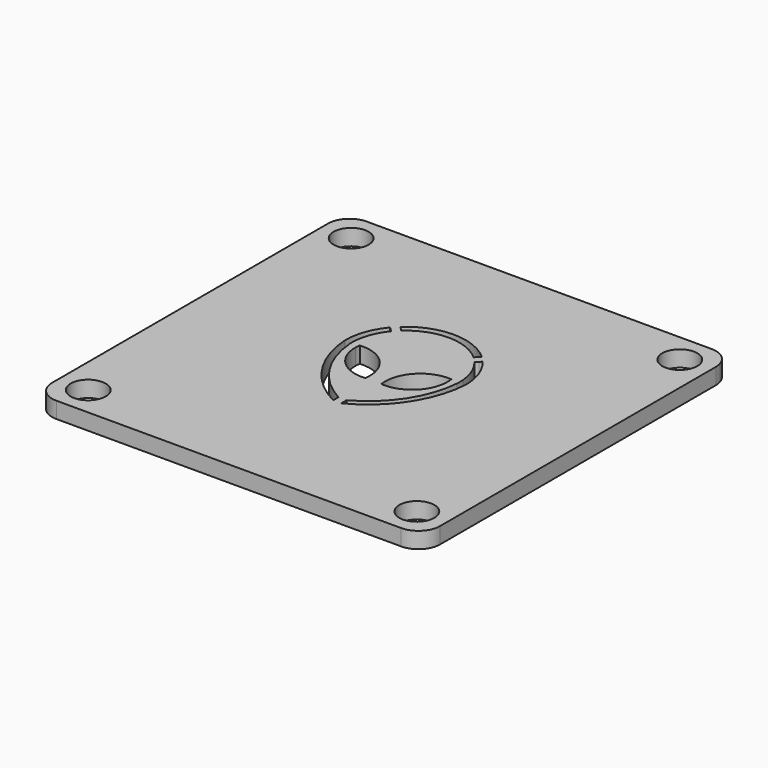
from build123d import *

# Parameters (mm, degrees)
F0_W        = 36
F0_H        = 36
F0_R        = 1.625
F1_DEPTH    = 1.5
F2_R        = 2
F3_T1_DEPTH = 3.5843159378
F3_T3_DEPTH = 3.5765382717


# Not quite as in the source:
# - a fillet or chamfer that OpenCascade refuses, or shapes differently, is made with other operations: its cross-section is extruded or revolved along the edge and cut away or added


with BuildPart() as f1:
    # F0 (on Top) → F1 (new body)
    with BuildSketch(Plane.XY):
        with Locations((18, -18)):
            Rectangle(F0_W, F0_H)
        with Locations((2.75, -33.25)):
            Circle(F0_R, mode=Mode.SUBTRACT)
        with Locations((33.25, -33.25)):
            Circle(F0_R, mode=Mode.SUBTRACT)
        with BuildLine():
            ThreePointArc((21.7779175478, -11.3763919814), (22.046238649, -11.6387988402), (22.2963811606, -11.918588577))
            ThreePointArc((22.2963811606, -11.918588577), (23.2607600241, -13.5926773143), (23.5988556823, -15.4948579101))
            ThreePointArc((23.5988556823, -15.4948579101), (22.0425607669, -20.1541714045), (18.3719356765, -23.4187950503))
            ThreePointArc((18.3719356765, -23.4187950503), (18.1854087753, -23.510113363), (17.9969356765, -23.5973441498))
            ThreePointArc((17.9969356765, -23.5973441498), (17.8078713111, -23.5092095417), (17.6207740645, -23.4169725439))
            ThreePointArc((17.6207740645, -23.4169725439), (13.9590716003, -20.150973111), (12.3987158352, -15.4990802577))
            ThreePointArc((12.3987158352, -15.4990802577), (12.7360960776, -13.5946679159), (13.7011902766, -11.9185996051))
            ThreePointArc((13.7011902766, -11.9185996051), (13.9513320879, -11.638809208), (14.2196525358, -11.3764016446))
            ThreePointArc((14.2196525358, -11.3764016446), (17.9987831657, -9.9089991809), (21.7779175478, -11.3763919814))
        make_face(mode=Mode.SUBTRACT)
        with Locations((2.75, -2.75)):
            Circle(F0_R, mode=Mode.SUBTRACT)
        with Locations((33.25, -2.75)):
            Circle(F0_R, mode=Mode.SUBTRACT)
        with BuildLine():
            ThreePointArc((18.3719356765, -22.8064015707), (21.6418869825, -19.7559203536), (22.9988556823, -15.4948579101))
            ThreePointArc((22.9988556823, -15.4948579101), (22.7058670076, -13.8225937813), (21.8702080342, -12.3447630196))
            ThreePointArc((21.8702080342, -12.3447630196), (21.6219028277, -12.0632376766), (21.3531767506, -11.8011340904))
            ThreePointArc((21.3531767506, -11.8011340904), (17.9987795183, -10.508999181), (14.644381672, -11.8011324963))
            ThreePointArc((14.644381672, -11.8011324963), (14.3756554704, -12.0632359548), (14.12735013, -12.3447611798))
            ThreePointArc((14.12735013, -12.3447611798), (13.2916900536, -13.8225926629), (12.9987009782, -15.4948579101))
            ThreePointArc((12.9987009782, -15.4948579101), (14.3541308063, -19.7551514484), (17.6219356765, -22.8061746181))
            ThreePointArc((17.6219356765, -22.8061746181), (17.8082968783, -22.9039932616), (17.9969356765, -22.9973441498))
            ThreePointArc((17.9969356765, -22.9973441498), (18.1855728443, -22.9041061909), (18.3719356765, -22.8064015707))
        make_face()
        with BuildLine():
            ThreePointArc((13.7508900496, -15.5000002377), (16.4147091349, -16.5221024247), (17.2508900496, -19.2500002377))
            ThreePointArc((17.2508900496, -19.2500002377), (14.7355024037, -18.3769724477), (13.7124911572, -15.9187616104))
            ThreePointArc((13.7124911572, -15.9187616104), (13.7249235892, -15.7087604135), (13.7508900496, -15.5000002377))
        make_face(mode=Mode.SUBTRACT)
        with BuildLine():
            ThreePointArc((18.7512718965, -19.25059231), (19.5857343833, -16.5222080691), (22.2488645533, -15.4984180975))
            ThreePointArc((22.2488645533, -15.4984180975), (21.4144020665, -18.2268023385), (18.7512718965, -19.25059231))
        make_face(mode=Mode.SUBTRACT)
        with BuildLine():
            Line((18.3719356765, -23.2973441498), (18.3719356765, -22.8064015707))
            ThreePointArc((18.3719356765, -22.8064015707), (18.1855728443, -22.9041061909), (17.9969356765, -22.9973441498))
            ThreePointArc((17.9969356765, -22.9973441498), (17.8082968783, -22.9039932616), (17.6219356765, -22.8061746181))
            Line((17.6219356765, -22.8061746181), (17.6219356765, -23.2973441498))
            Line((17.6219356765, -23.2973441498), (17.6207740645, -23.4169725439))
            ThreePointArc((17.6207740645, -23.4169725439), (17.8078713111, -23.5092095417), (17.9969356765, -23.5973441498))
            ThreePointArc((17.9969356765, -23.5973441498), (18.1854087753, -23.510113363), (18.3719356765, -23.4187950503))
            Line((18.3719356765, -23.4187950503), (18.3719356765, -23.2973441498))
        make_face()
        with BuildLine():
            ThreePointArc((21.3531767506, -11.8011340904), (21.6219028277, -12.0632376766), (21.8702080342, -12.3447630196))
            Line((21.8702080342, -12.3447630196), (22.1000614519, -12.114908892))
            Line((22.1000614519, -12.114908892), (22.2963811606, -11.918588577))
            ThreePointArc((22.2963811606, -11.918588577), (22.046238649, -11.6387988402), (21.7779175478, -11.3763919814))
            Line((21.7779175478, -11.3763919814), (21.5697305471, -11.5845796251))
            Line((21.5697305471, -11.5845796251), (21.3531767506, -11.8011340904))
        make_face()
        with BuildLine():
            ThreePointArc((14.12735013, -12.3447611798), (14.3756554704, -12.0632359548), (14.644381672, -11.8011324963))
            Line((14.644381672, -11.8011324963), (14.4278279784, -11.584577928))
            Line((14.4278279784, -11.584577928), (14.2196525358, -11.3764016446))
            ThreePointArc((14.2196525358, -11.3764016446), (13.9513320879, -11.638809208), (13.7011902766, -11.9185996051))
            Line((13.7011902766, -11.9185996051), (13.8974968216, -12.114906943))
            Line((13.8974968216, -12.114906943), (14.12735013, -12.3447611798))
        make_face()
    extrude(amount=F1_DEPTH)

    # F2
    f2_edges = [f1.edges().sort_by_distance(p)[0] for p in [
        (36, -36, 0.75),
        (0, -36, 0.75),
        (36, 0, 0.75),
        (0, 0, 0.75),
    ]]
    fillet(f2_edges, radius=F2_R)

    # F3: fillet of radius 4 on 2 edges, made by hand

    # F3_s2 → F3_t1 (cut)
    with BuildSketch(Plane.XY.offset(-1.0421579689)):
        with BuildLine():
            ThreePointArc((22.982065791, -15.7463315161), (22.9951448823, -15.4123328014), (22.980292521, -15.0784082419))
            ThreePointArc((22.980292521, -15.0784082419), (22.9939159673, -15.2864395382), (22.9988556823, -15.4948579101))
            ThreePointArc((22.9988556823, -15.4948579101), (22.9913576348, -15.6206545954), (22.982065791, -15.7463315161))
        make_face()
    extrude(amount=F3_T1_DEPTH, mode=Mode.SUBTRACT)

    # F3_s4 → F3_t3 (cut)
    with BuildSketch(Plane.XY.offset(-1.0382691359)):
        with BuildLine():
            ThreePointArc((13.0171302774, -15.0799593578), (13.0023850075, -15.4126416016), (13.0153633645, -15.745397459))
            ThreePointArc((13.0153633645, -15.745397459), (13.0061419392, -15.6201868903), (12.9987009782, -15.4948579101))
            ThreePointArc((12.9987009782, -15.4948579101), (13.0036060893, -15.2872172094), (13.0171302774, -15.0799593578))
        make_face()
    extrude(amount=F3_T3_DEPTH, mode=Mode.SUBTRACT)


solid = f1.part
